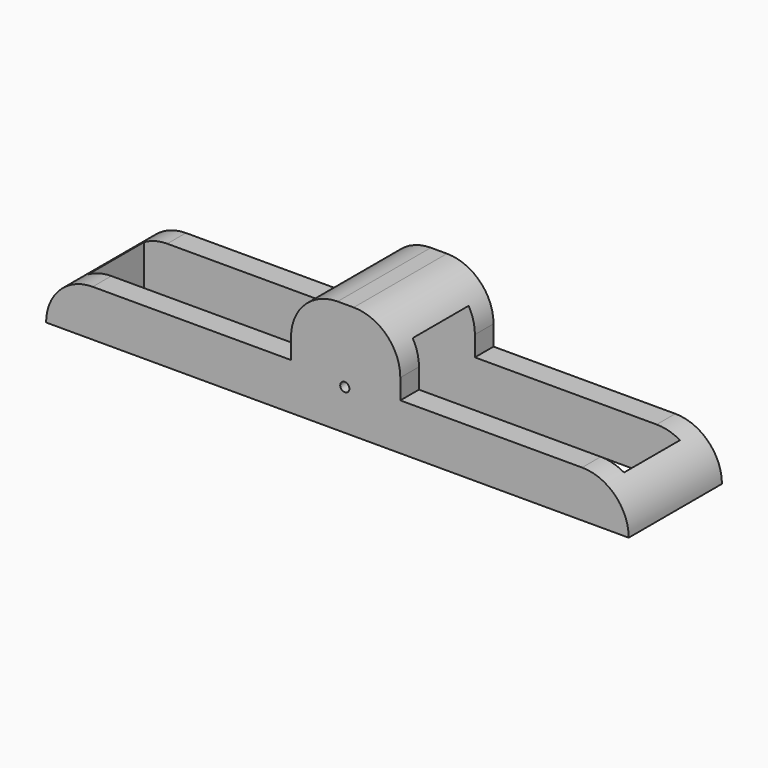
from build123d import *

# Parameters (mm, degrees)
F0_W        = 22.3517898379
F0_H        = 5.08
F0_W_2      = 24.1537776476
F0_W_3      = 6.0488656163
F0_H_2      = 4.7264951599
F0_W_4      = 5.8655668981
F1_DEPTH    = 7.62
F2_T        = 2.54
F3_R        = 0.5
F4_DEPTH    = 8.10174
F6_T1_DEPTH = 38.1
F6_T3_DEPTH = 38.1
F6_T5_DEPTH = 38.1
F6_T7_DEPTH = 38.1
F7_DEPTH    = 7.36236


# Not quite as in the source:
# - a fillet or chamfer that OpenCascade refuses, or shapes differently, is made with other operations: its cross-section is extruded or revolved along the edge and cut away or added
# - a feature of the source that left no trace in its solid (it failed there, or was rolled back) is left out


with BuildPart() as f1:
    # F0 (on Front) → F1 (new body)
    with BuildSketch(Plane.XZ):
        Polygon((-5.8655668981, 0), (0, 0), (6.0488656163, 0), (6.0488656163, 5.08), (0, 5.08), (-5.8655668981, 5.08), align=None)
        with Locations((17.2247605353, 2.54)):
            Rectangle(F0_W, F0_H)
        with Locations((-17.942455722, 2.54)):
            Rectangle(F0_W_2, F0_H)
        with Locations((3.0244328082, 7.4432475799)):
            Rectangle(F0_W_3, F0_H_2)
        with Locations((-2.9327834491, 7.4432475799)):
            Rectangle(F0_W_4, F0_H_2)
    extrude(amount=F1_DEPTH)

    # F2
    f2_openings = [f1.faces().sort_by_distance(p)[0] for p in [
        (-17.942456, -3.81, 5.08),
        (-0.809345, -3.81, 0),
        (17.224761, -3.81, 5.08),
        (6.048866, -3.81, 7.443248),
        (-5.865567, -3.81, 7.443248),
    ]]
    offset(amount=F2_T, openings=f2_openings, kind=Kind.INTERSECTION)

    # F3 (on face) → F4 (cut)
    with BuildSketch(Plane.XZ.offset(10.16)):
        with Locations((0, 4.3936586007)):
            Circle(F3_R)
    extrude(amount=-F4_DEPTH, mode=Mode.SUBTRACT)

    # F6: fillet of radius 5.08 on 6 edges, made by hand

    # F6_s2 → F6_t1 (cut)
    with BuildSketch(Plane.XZ.offset(-15.24)):
        with BuildLine():
            ThreePointArc((25.8606554542, 5.08), (29.4527579027, 3.5921024484), (30.9406554542, 0))
            Line((30.9406554542, 0), (31.0422554542, 0))
            Line((31.0422554542, 0), (31.0422554542, 5.1816))
            Line((31.0422554542, 5.1816), (25.8606554542, 5.1816))
            Line((25.8606554542, 5.1816), (25.8606554542, 5.08))
        make_face()
    extrude(amount=F6_T1_DEPTH, mode=Mode.SUBTRACT)

    # F6_s4 → F6_t3 (cut)
    with BuildSketch(Plane.XZ.offset(-15.24)):
        with BuildLine():
            ThreePointArc((-27.4793445458, 5.08), (-31.0714469942, 3.5921024484), (-32.5593445458, 0))
            Line((-32.5593445458, 0), (-32.6609445458, 0))
            Line((-32.6609445458, 0), (-32.6609445458, 5.1816))
            Line((-32.6609445458, 5.1816), (-27.4793445458, 5.1816))
            Line((-27.4793445458, 5.1816), (-27.4793445458, 5.08))
        make_face()
    extrude(amount=F6_T3_DEPTH, mode=Mode.SUBTRACT)

    # F6_s6 → F6_t5 (cut)
    with BuildSketch(Plane.XZ.offset(-15.24)):
        with BuildLine():
            ThreePointArc((6.0488656163, 7.2664951599), (4.5609680647, 10.8585976083), (0.9688656163, 12.3464951599))
            Line((0.9688656163, 12.3464951599), (0.9688656163, 12.4480951599))
            Line((0.9688656163, 12.4480951599), (6.1504656163, 12.4480951599))
            Line((6.1504656163, 12.4480951599), (6.1504656163, 7.2664951599))
            Line((6.1504656163, 7.2664951599), (6.0488656163, 7.2664951599))
        make_face()
    extrude(amount=F6_T5_DEPTH, mode=Mode.SUBTRACT)

    # F6_s8 → F6_t7 (cut)
    with BuildSketch(Plane.XZ.offset(-15.24)):
        with BuildLine():
            ThreePointArc((-5.8655668981, 7.2664951599), (-4.3776693466, 10.8585976083), (-0.7855668981, 12.3464951599))
            Line((-0.7855668981, 12.3464951599), (-0.7855668981, 12.4480951599))
            Line((-0.7855668981, 12.4480951599), (-5.9671668981, 12.4480951599))
            Line((-5.9671668981, 12.4480951599), (-5.9671668981, 7.2664951599))
            Line((-5.9671668981, 7.2664951599), (-5.8655668981, 7.2664951599))
        make_face()
    extrude(amount=F6_T7_DEPTH, mode=Mode.SUBTRACT)

    # F3 (on face) → F7 (cut)
    with BuildSketch(Plane.XZ.offset(10.16)):
        with Locations((0, 4.3936586007)):
            Circle(F3_R)
    extrude(amount=-F7_DEPTH, mode=Mode.SUBTRACT)


solid = f1.part
